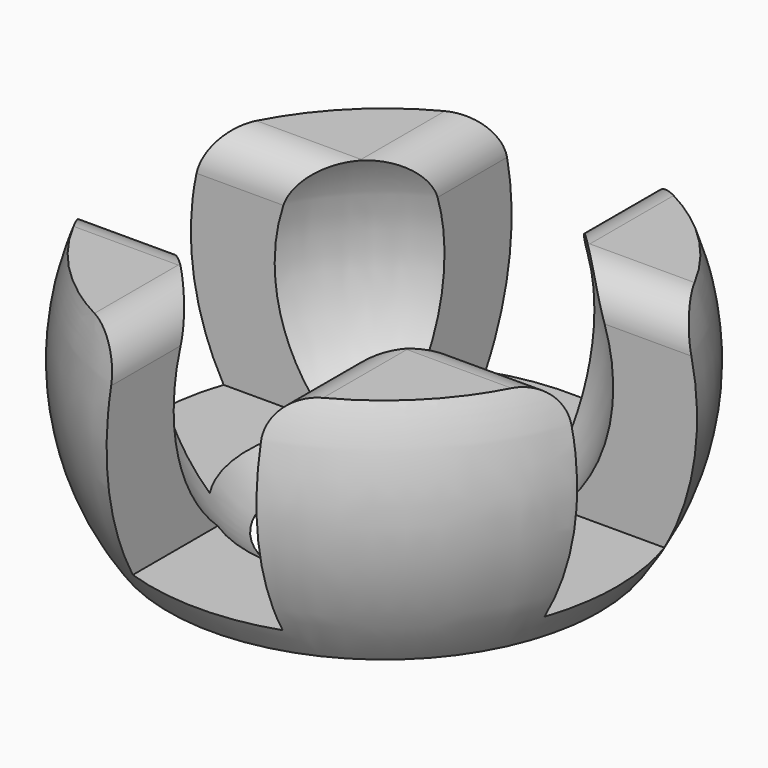
from build123d import *

# Parameters (mm, degrees)
F2_W         = 15
F2_H         = 7
F3_DEPTH     = 12.5
F5_DEPTH     = 5.5
F6_W         = 14
F6_H         = 3.8
F7_DEPTH     = 12.5
F8_T1_DEPTH  = 7.385872422
F8_T3_DEPTH  = 7.3858724269
F8_T5_DEPTH  = 7.3858724206
F8_T7_DEPTH  = 7.3858724234
F8_T9_DEPTH  = 7.3858724333
F8_T11_DEPTH = 7.3858724191
F8_T13_DEPTH = 7.3858723897


# Not quite as in the source:
# - a fillet or chamfer that OpenCascade refuses, or shapes differently, is made with other operations: its cross-section is extruded or revolved along the edge and cut away or added


with BuildPart() as f1:
    # F0 (on Front) → F1 (revolve)
    with BuildSketch(Plane.XZ):
        with BuildLine():
            Line((0, 2.0000641001), (0, 0))
            ThreePointArc((0, 0), (6.6945200517, 6.6498509731), (0, 13.2997019463))
            Line((0, 13.2997019463), (0, 11.2996378462))
            ThreePointArc((0, 11.2996378462), (4.6945200517, 6.6498509731), (0, 2.0000641001))
        make_face()
    revolve(axis=Axis((0, 0, 10.4240386703), (0, 0, -1)))

    # F2 (on Front) → F3 (cut, symmetric)
    with BuildSketch(Plane.XZ):
        with Locations((0, 12.5)):
            Rectangle(F2_W, F2_H)
    extrude(amount=F3_DEPTH, both=True, mode=Mode.SUBTRACT)

    # F4 (on face) → F5 (cut)
    with BuildSketch(Plane.XY.offset(9)):
        Polygon((-1.9, 1.9), (-7, 1.9), (-7, -1.9), (-1.9, -1.9), (-1.9, -7), (1.9, -7), (1.9, -1.9), (7, -1.9), (7, 1.9), (1.9, 1.9), (1.9, 7), (-1.9, 7), align=None)
    extrude(amount=-F5_DEPTH, mode=Mode.SUBTRACT)

    # F6 (on Front) → F7 (cut, symmetric)
    with BuildSketch(Plane.XZ):
        with Locations((0, 0.9)):
            Rectangle(F6_W, F6_H)
    extrude(amount=F7_DEPTH, both=True, mode=Mode.SUBTRACT)

    # F8: fillet of radius 1 on 8 edges, made by hand

    # F8_s2 → F8_t1 (cut)
    with BuildSketch(Plane.YZ.offset(1.0844867834)):
        with BuildLine():
            ThreePointArc((2.9, 9), (2.1928932188, 8.7071067812), (1.9, 8))
            Line((1.9, 8), (1.9, 9))
            Line((1.9, 9), (2.9, 9))
        make_face()
    extrude(amount=F8_T1_DEPTH, mode=Mode.SUBTRACT)

    # F8_s4 → F8_t3 (cut)
    with BuildSketch(Plane.XZ.offset(-8.4703592108)):
        with BuildLine():
            ThreePointArc((2.9, 9), (2.1928932188, 8.7071067812), (1.9, 8))
            Line((1.9, 8), (1.9, 9))
            Line((1.9, 9), (2.9, 9))
        make_face()
    extrude(amount=F8_T3_DEPTH, mode=Mode.SUBTRACT)

    # F8_s6 → F8_t5 (cut)
    with BuildSketch(Plane.XZ.offset(-8.4703592054)):
        with BuildLine():
            ThreePointArc((-1.9, 8), (-2.1928932188, 8.7071067812), (-2.9, 9))
            Line((-2.9, 9), (-1.9, 9))
            Line((-1.9, 9), (-1.9, 8))
        make_face()
    extrude(amount=F8_T5_DEPTH, mode=Mode.SUBTRACT)

    # F8_s8 → F8_t7 (cut)
    with BuildSketch(Plane.YZ.offset(-8.4703592108)):
        with BuildLine():
            ThreePointArc((2.9, 9), (2.1928932188, 8.7071067812), (1.9, 8))
            Line((1.9, 8), (1.9, 9))
            Line((1.9, 9), (2.9, 9))
        make_face()
    extrude(amount=F8_T7_DEPTH, mode=Mode.SUBTRACT)

    # F8_s10 → F8_t9 (cut)
    with BuildSketch(Plane.YZ.offset(-8.4703592057)):
        with BuildLine():
            ThreePointArc((-1.9, 8), (-2.1928932188, 8.7071067812), (-2.9, 9))
            Line((-2.9, 9), (-1.9, 9))
            Line((-1.9, 9), (-1.9, 8))
        make_face()
    extrude(amount=F8_T9_DEPTH, mode=Mode.SUBTRACT)

    # F8_s12 → F8_t11 (cut)
    with BuildSketch(Plane.XZ.offset(1.0844867941)):
        with BuildLine():
            ThreePointArc((-2.9, 9), (-2.1928932188, 8.7071067812), (-1.9, 8))
            Line((-1.9, 8), (-1.9, 9))
            Line((-1.9, 9), (-2.9, 9))
        make_face()
        with BuildLine():
            ThreePointArc((1.9, 8), (2.1928932188, 8.7071067812), (2.9, 9))
            Line((2.9, 9), (1.9, 9))
            Line((1.9, 9), (1.9, 8))
        make_face()
    extrude(amount=F8_T11_DEPTH, mode=Mode.SUBTRACT)

    # F8_s14 → F8_t13 (cut)
    with BuildSketch(Plane.YZ.offset(1.0844868043)):
        with BuildLine():
            ThreePointArc((-2.9, 9), (-2.1928932188, 8.7071067812), (-1.9, 8))
            Line((-1.9, 8), (-1.9, 9))
            Line((-1.9, 9), (-2.9, 9))
        make_face()
    extrude(amount=F8_T13_DEPTH, mode=Mode.SUBTRACT)


solid = f1.part
